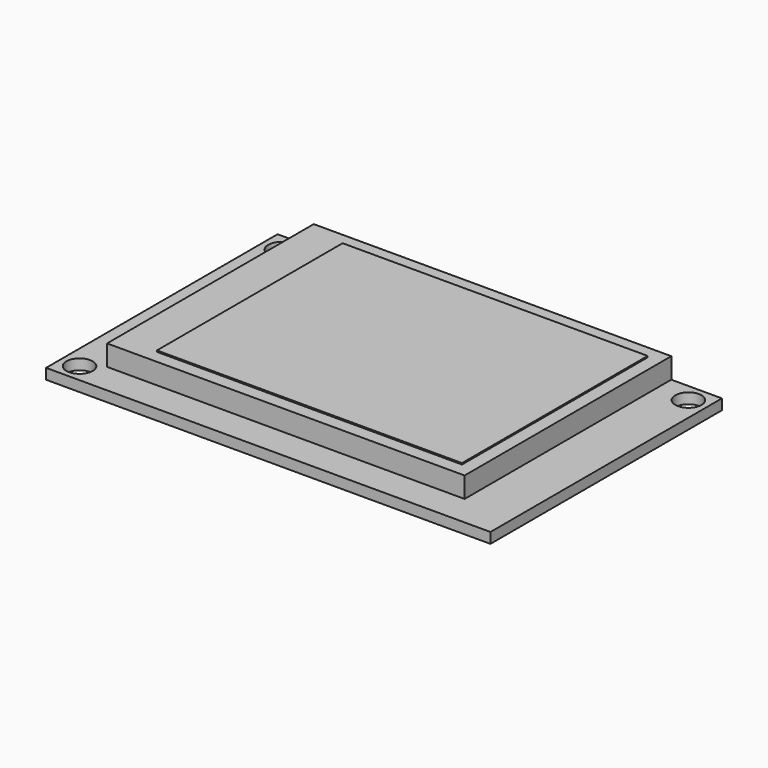
from build123d import *

# Parameters (mm, degrees)
F0_W     = 86
F0_H     = 56
F0_R     = 2.54
F1_DEPTH = 2.032
F2_W     = 69.2
F2_H     = 50
F3_DEPTH = 4
F5_W     = 59.04
F5_H     = 44.92
F6_DEPTH = 0.254


# Not quite as in the source:
# - a feature of the source that left no trace in its solid (it failed there, or was rolled back) is left out


with BuildPart() as f1:
    # F0 (on Top) → F1 (new body)
    with BuildSketch(Plane.XY):
        Rectangle(F0_W, F0_H)
        with Locations((-39.4, -24.4)):
            Circle(F0_R, mode=Mode.SUBTRACT)
        with Locations((-39.4, 24.4)):
            Circle(F0_R, mode=Mode.SUBTRACT)
        with Locations((39.4, 24.4)):
            Circle(F0_R, mode=Mode.SUBTRACT)
    extrude(amount=-F1_DEPTH)


with BuildPart() as f3:
    # F2 (on Top) → F3 (new body)
    with BuildSketch(Plane.XY):
        with Locations((-1.4, 3)):
            Rectangle(F2_W, F2_H)
    extrude(amount=F3_DEPTH)

    # F5 (on face) → F6 (join)
    with BuildSketch(Plane.XY.offset(4)):
        with Locations((1.14, 3)):
            Rectangle(F5_W, F5_H)
    extrude(amount=F6_DEPTH)


solid = Compound([f1.part, f3.part])
